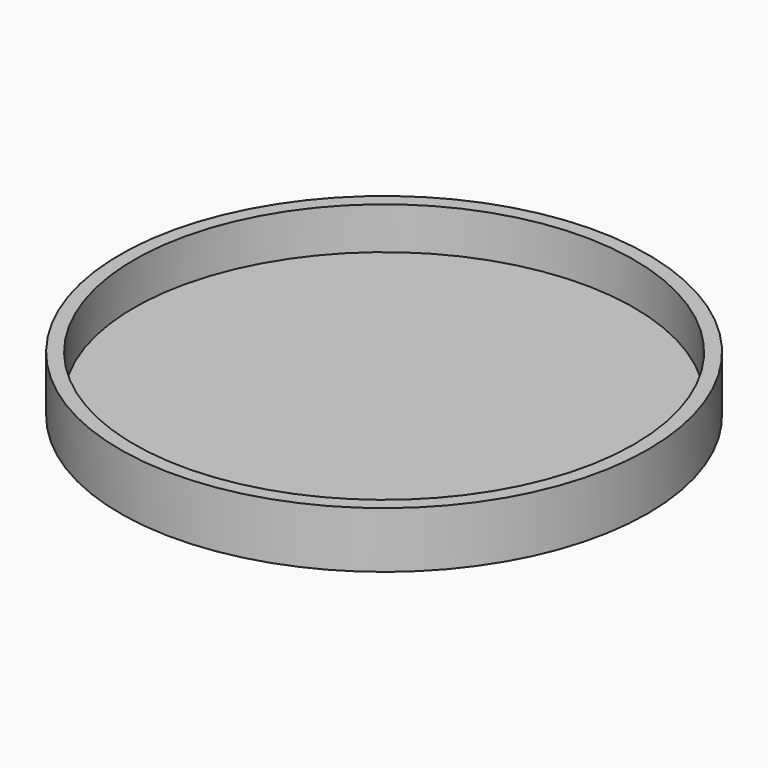
from build123d import *

# Parameters (mm, degrees)
F0_R     = 59.69
F0_R_2   = 56.515
F1_DEPTH = 12.7
F2_DEPTH = 3.175
F3_R     = 21.425
F3_R_2   = 18.25
F4_DEPTH = 12.7


# Not quite as in the source:
# - a feature names something its author has since deleted; it is built from what else it names


with BuildPart() as f1:
    # F0 (on Top) → F1 (new body)
    with BuildSketch(Plane.XY):
        Circle(F0_R)
        Circle(F0_R_2, mode=Mode.SUBTRACT)
    extrude(amount=F1_DEPTH)

    # F0 (on Top) → F2 (join)
    with BuildSketch(Plane.XY):
        Circle(F0_R_2)
    extrude(amount=F2_DEPTH)

    # F3 (on face) → F4 (join)
    with BuildSketch(Plane.XY):
        Circle(F3_R)
        Circle(F3_R_2, mode=Mode.SUBTRACT)
    extrude(amount=-F4_DEPTH)


solid = f1.part
